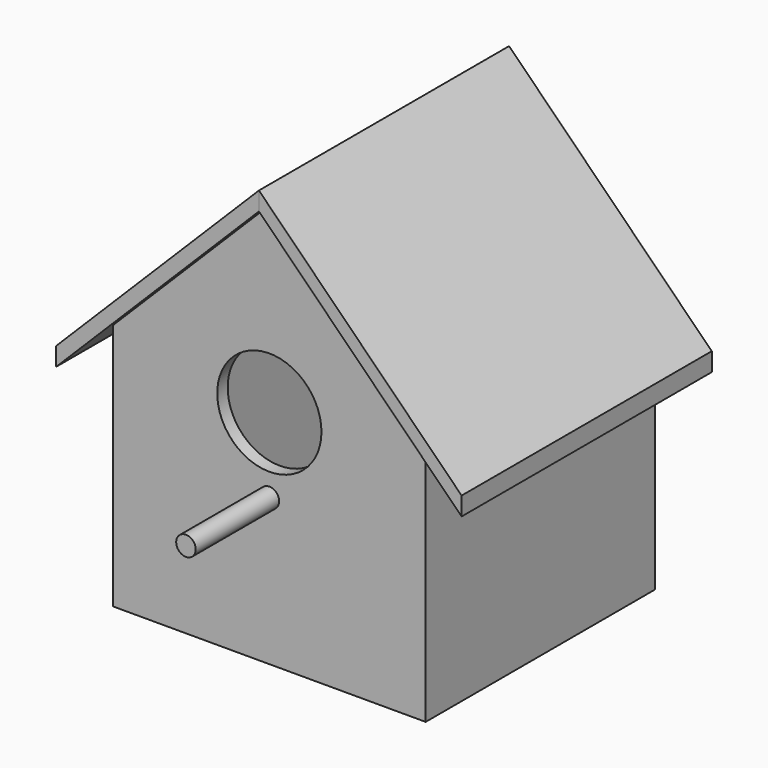
from build123d import *

# Parameters (mm, degrees)
F0_W           = 152.4
F0_H           = 6.35
F1_DEPTH       = 139.7
F2_SIZE2       = 6.34999
F2_SIZE        = 6.34999
F3_W           = 6.35
F3_H           = 127
F4_DEPTH       = 139.7
F5_SIZE2       = 6.34999
F5_SIZE        = 6.34999
F5_2_SIZE2     = 6.34999
F5_2_SIZE      = 6.34999
F7_R           = 4.7625
F7_R_2         = 25.4
F8_DEPTH       = 6.35
F10_DEPTH      = 6.35
F11_SIZE2      = 6.34999
F11_SIZE       = 6.34999
F11_2_SIZE2    = 6.34999
F11_2_SIZE     = 6.34999
F13_DEPTH      = 6.35
F13_DEPTH_BACK = 146.05
F16_DEPTH      = 50.8


# Not quite as in the source:
# - a fillet or chamfer is up to 0.001 mm smaller than in the source, because OpenCascade refuses the exact size


with BuildPart() as f1:
    # F0 (on Front) → F1 (new body)
    with BuildSketch(Plane.XZ):
        with Locations((0, 3.175)):
            Rectangle(F0_W, F0_H)
    extrude(amount=-F1_DEPTH)

    # F2 (size 6.35 and 6.35 in the source; OpenCascade refuses exactly that, so slightly less here)
    f2_edges = [f1.edges().sort_by_distance(p)[0] for p in [
        (76.2, 69.85, 6.35),
        (-76.2, 69.85, 6.35),
        (0, 0, 6.35),
        (0, 139.7, 6.35),
    ]]
    chamfer(f2_edges, length=F2_SIZE, length2=F2_SIZE2)


with BuildPart() as f4:
    # F3 (on Front) → F4 (new body)
    with BuildSketch(Plane.XZ):
        with Locations((-73.025, 63.5)):
            Rectangle(F3_W, F3_H)
    extrude(amount=-F4_DEPTH)

    # F5 (size 6.35 and 6.35 in the source; OpenCascade refuses exactly that, so slightly less here)
    f5_edges = [f4.edges().sort_by_distance(p)[0] for p in [
        (-69.85, 139.7, 63.5),
        (-69.85, 69.85, 0),
        (-69.85, 0, 63.5),
    ]]
    chamfer(f5_edges, length=F5_SIZE, length2=F5_SIZE2)


with BuildPart() as f4b:
    # F3 (on Front) → F4, piece 2 (new body)
    with BuildSketch(Plane.XZ):
        with Locations((73.025, 63.5)):
            Rectangle(F3_W, F3_H)
    extrude(amount=-F4_DEPTH)

    # F5#2 (size 6.35 and 6.35 in the source; OpenCascade refuses exactly that, so slightly less here)
    f5_2_edges = [f4b.edges().sort_by_distance(p)[0] for p in [
        (69.85, 0, 63.5),
        (69.85, 69.85, 0),
        (69.85, 139.7, 63.5),
    ]]
    chamfer(f5_2_edges, length=F5_2_SIZE, length2=F5_2_SIZE2)


with BuildPart() as f8:
    # F7 (on Front) → F8 (new body)
    with BuildSketch(Plane.XZ):
        Polygon((76.2, 120.65), (0, 196.85), (-76.2, 120.65), (-76.2, 0), (76.2, 0), align=None)
        with Locations((0, 71.4375)):
            Circle(F7_R, mode=Mode.SUBTRACT)
        with Locations((0, 107.95)):
            Circle(F7_R_2, mode=Mode.SUBTRACT)
    extrude(amount=-F8_DEPTH)

    # F11 (size 6.35 and 6.35 in the source; OpenCascade refuses exactly that, so slightly less here)
    f11_edges = [f8.edges().sort_by_distance(p)[0] for p in [
        (76.2, 6.35, 60.325),
        (0, 6.35, 0),
        (-76.2, 6.35, 60.325),
    ]]
    chamfer(f11_edges, length=F11_SIZE, length2=F11_SIZE2)


with BuildPart() as f10:
    # F9 (on offset) → F10 (new body)
    with BuildSketch(Plane.XZ.offset(-139.7)):
        Polygon((76.2, 120.65), (0, 196.85), (-76.2, 120.65), (-76.2, 0), (76.2, 0), align=None)
    extrude(amount=F10_DEPTH)

    # F11#2 (size 6.35 and 6.35 in the source; OpenCascade refuses exactly that, so slightly less here)
    f11_2_edges = [f10.edges().sort_by_distance(p)[0] for p in [
        (-76.2, 133.35, 60.325),
        (0, 133.35, 0),
        (76.2, 133.35, 60.325),
    ]]
    chamfer(f11_2_edges, length=F11_2_SIZE, length2=F11_2_SIZE2)


with BuildPart() as f13:
    # F12 (on Front) → F13 (new body, two sides)
    with BuildSketch(Plane.XZ) as f13_sk:
        Polygon((-98.7828173318, 98.0671826682), (0, 196.85), (0, 205.8302561211), (-98.7828173318, 107.0474387893), align=None)
    extrude(amount=F13_DEPTH)
    extrude(f13_sk.sketch, amount=-F13_DEPTH_BACK)


with BuildPart() as f14_1:
    # F14: instance of F13
    add(f13.part.mirror(Plane.YZ))


with BuildPart() as f4_1:
    add(f4.part)

    # F15: cut F13, F14_1
    add(f13.part, mode=Mode.SUBTRACT)
    add(f14_1.part, mode=Mode.SUBTRACT)


with BuildPart() as f4b_1:
    add(f4b.part)

    # F15: cut F13, F14_1
    add(f13.part, mode=Mode.SUBTRACT)
    add(f14_1.part, mode=Mode.SUBTRACT)


with BuildPart() as f16:
    # F7 (on Front) → F16 (new body)
    with BuildSketch(Plane.XZ):
        with Locations((0, 71.4375)):
            Circle(F7_R)
    extrude(amount=F16_DEPTH)


solid = Compound([f1.part, f8.part, f10.part, f13.part, f14_1.part, f4_1.part, f4b_1.part, f16.part])
